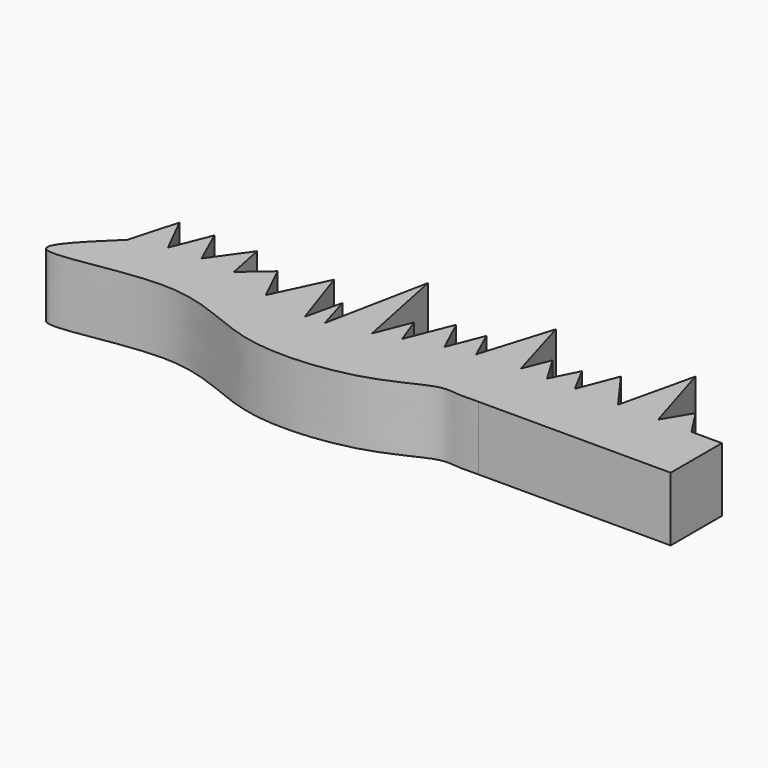
from build123d import *

# Parameters (mm, degrees)
F1_DEPTH = 12.7


# Not quite as in the source:
# - a feature names something its author has since deleted; it is built from what else it names


with BuildPart() as f1:
    # F0 (on Top) → F1 (new body)
    with BuildSketch(Plane.XY):
        with BuildLine():
            Line((29.1566601902, 1.7817904405), (29.1566601902, 14.4817904405))
            Line((29.1566601902, 14.4817904405), (23.1322348118, 14.4817904405))
            Line((23.1322348118, 14.4817904405), (16.5050514042, 14.4817904405))
            Line((16.5050514042, 14.4817904405), (8.552428335, 14.4817904405))
            Line((8.552428335, 14.4817904405), (0, 14.4817904405))
            Line((0, 14.4817904405), (-5.4972041398, 14.4817904405))
            Line((-5.4972041398, 14.4817904405), (-8.9433398098, 14.4817904405))
            add(Edge.make_bspline(
                [(-8.9433398098, 14.4817904405), (-10.7573023584, 14.5540929372), (-13.6536245903, 14.6695370673), (-17.5443018447, 14.2319983354), (-19.1478505954, 13.9692945078)],
                knots=[0, 0, 0, 0, 0.1219531365, 0.1947204372, 0.1947204372, 0.1947204372, 0.1947204372], degree=3))
            add(Edge.make_bspline(
                [(-19.1478505954, 13.9692945078), (-20.7855145388, 13.7010017066), (-22.5792086961, 13.3292483099), (-24.5403655562, 12.8306326712)],
                knots=[0.1947204372, 0.1947204372, 0.1947204372, 0.1947204372, 0.2690358483, 0.2690358483, 0.2690358483, 0.2690358483], degree=3))
            add(Edge.make_bspline(
                [(-24.5403655562, 12.8306326712), (-25.4054556528, 12.6106872606), (-27.5608275588, 12.0233152228), (-29.9097113738, 11.2820530364), (-31.3234997305, 10.8352217448)],
                knots=[0.2690358483, 0.2690358483, 0.2690358483, 0.2690358483, 0.3018172782, 0.3477460441, 0.3477460441, 0.3477460441, 0.3477460441], degree=3))
            add(Edge.make_bspline(
                [(-31.3234997305, 10.8352217448), (-32.8813721767, 10.3428523218), (-34.4916669077, 9.8331294404), (-36.1239915531, 9.3570380081)],
                knots=[0.3477460441, 0.3477460441, 0.3477460441, 0.3477460441, 0.3983555703, 0.3983555703, 0.3983555703, 0.3983555703], degree=3))
            add(Edge.make_bspline(
                [(-36.1239915531, 9.3570380081), (-38.7371673177, 8.5948669557), (-41.406802576, 7.9188884572), (-44.0082018162, 7.5382862352)],
                knots=[0.3983555703, 0.3983555703, 0.3983555703, 0.3983555703, 0.4793759651, 0.4793759651, 0.4793759651, 0.4793759651], degree=3))
            add(Edge.make_bspline(
                [(-44.0082018162, 7.5382862352), (-45.2733883847, 7.3531809228), (-46.5224347573, 7.2379423921), (-47.7409961664, 7.2166347961)],
                knots=[0.4793759651, 0.4793759651, 0.4793759651, 0.4793759651, 0.518780111, 0.518780111, 0.518780111, 0.518780111], degree=3))
            add(Edge.make_bspline(
                [(-47.7409961664, 7.2166347961), (-48.61023628, 7.2014353839), (-51.8736517816, 7.3260381182), (-54.8343256873, 8.2766625789), (-57.0016363215, 9.090849647)],
                knots=[0.518780111, 0.518780111, 0.518780111, 0.518780111, 0.5468883902, 0.6262253297, 0.6262253297, 0.6262253297, 0.6262253297], degree=3))
            add(Edge.make_bspline(
                [(-57.0016363215, 9.090849647), (-59.8222284032, 10.150452992), (-62.6109209229, 11.4001772385), (-65.6900354035, 12.0947333053)],
                knots=[0.6262253297, 0.6262253297, 0.6262253297, 0.6262253297, 0.7294764002, 0.7294764002, 0.7294764002, 0.7294764002], degree=3))
            add(Edge.make_bspline(
                [(-65.6900354035, 12.0947333053), (-67.0336130762, 12.397804214), (-69.2092078019, 12.7047556683), (-71.5833285763, 12.6062540598), (-72.4382368268, 12.5328440974)],
                knots=[0.7294764002, 0.7294764002, 0.7294764002, 0.7294764002, 0.7745302084, 0.7995461596, 0.7995461596, 0.7995461596, 0.7995461596], degree=3))
            add(Edge.make_bspline(
                [(-72.4382368268, 12.5328440974), (-78.4000977285, 12.0209061386), (-85.6590909795, 9.2956107983), (-85.3310582144, 10.1307918098), (-85.2885097265, 10.2391215041)],
                knots=[0.7995461596, 0.7995461596, 0.7995461596, 0.7995461596, 0.9739995247, 1, 1, 1, 1], degree=3))
            add(Edge.make_bspline(
                [(-8.9433398098, 1.7817904405), (-10.3062057468, 1.7346839959), (-12.9857258176, 1.6420683833), (-17.1466296289, 2.4827049446), (-27.1606442527, -4.0355858357), (-51.6393795509, -6.6773487114), (-67.5806364014, 5.6865791664), (-100.6765031612, -4.5794896544), (-89.9229154748, 5.7761967552), (-85.2885097265, 10.2391215041)],
                knots=[0, 0, 0, 0, 0.0795605261, 0.1564233287, 0.2898559981, 0.4816905838, 0.6666516763, 0.8563389789, 1, 1, 1, 1], degree=3))
            Line((-8.9433398098, 1.7817904405), (29.1566601902, 1.7817904405))
        make_face()
        with BuildLine():
            Line((-82.6221928, 19.7822675109), (-85.2885097265, 10.2391215041))
            add(Edge.make_bspline(
                [(-72.4382368268, 12.5328440974), (-78.4000977285, 12.0209061386), (-85.6590909795, 9.2956107983), (-85.3310582144, 10.1307918098), (-85.2885097265, 10.2391215041)],
                knots=[0.7995461596, 0.7995461596, 0.7995461596, 0.7995461596, 0.9739995247, 1, 1, 1, 1], degree=3))
            Line((-72.4382368268, 12.5328440974), (-75.7119506598, 19.7822675109))
            Line((-75.7119506598, 19.7822675109), (-78.7689969505, 12.0947333053))
            Line((-78.7689969505, 12.0947333053), (-82.6221928, 19.7822675109))
        make_face()
        with BuildLine():
            Line((-67.2413259745, 19.7822675109), (-72.4382368268, 12.5328440974))
            add(Edge.make_bspline(
                [(-65.6900354035, 12.0947333053), (-67.0336130762, 12.397804214), (-69.2092078019, 12.7047556683), (-71.5833285763, 12.6062540598), (-72.4382368268, 12.5328440974)],
                knots=[0.7294764002, 0.7294764002, 0.7294764002, 0.7294764002, 0.7745302084, 0.7995461596, 0.7995461596, 0.7995461596, 0.7995461596], degree=3))
            Line((-65.6900354035, 12.0947333053), (-67.2413259745, 19.7822675109))
        make_face()
        with BuildLine():
            Line((-51.9719198346, 19.7822675109), (-57.0016363215, 9.090849647))
            add(Edge.make_bspline(
                [(-47.7409961664, 7.2166347961), (-48.61023628, 7.2014353839), (-51.8736517816, 7.3260381182), (-54.8343256873, 8.2766625789), (-57.0016363215, 9.090849647)],
                knots=[0.518780111, 0.518780111, 0.518780111, 0.518780111, 0.5468883902, 0.6262253297, 0.6262253297, 0.6262253297, 0.6262253297], degree=3))
            Line((-47.7409961664, 7.2166347961), (-51.9719198346, 19.7822675109))
        make_face()
        with BuildLine():
            Line((-46.0647791624, 14.4817904405), (-47.7409961664, 7.2166347961))
            add(Edge.make_bspline(
                [(-44.0082018162, 7.5382862352), (-45.2733883847, 7.3531809228), (-46.5224347573, 7.2379423921), (-47.7409961664, 7.2166347961)],
                knots=[0.4793759651, 0.4793759651, 0.4793759651, 0.4793759651, 0.518780111, 0.518780111, 0.518780111, 0.518780111], degree=3))
            Line((-44.0082018162, 7.5382862352), (-46.0647791624, 14.4817904405))
        make_face()
        with BuildLine():
            Line((-39.9164316104, 27.9997758427), (-44.0082018162, 7.5382862352))
            add(Edge.make_bspline(
                [(-36.1239915531, 9.3570380081), (-38.7371673177, 8.5948669557), (-41.406802576, 7.9188884572), (-44.0082018162, 7.5382862352)],
                knots=[0.3983555703, 0.3983555703, 0.3983555703, 0.3983555703, 0.4793759651, 0.4793759651, 0.4793759651, 0.4793759651], degree=3))
            Line((-36.1239915531, 9.3570380081), (-39.9164316104, 27.9997758427))
        make_face()
        with BuildLine():
            Line((-33.3588495851, 16.3105223328), (-36.1239915531, 9.3570380081))
            add(Edge.make_bspline(
                [(-31.3234997305, 10.8352217448), (-32.8813721767, 10.3428523218), (-34.4916669077, 9.8331294404), (-36.1239915531, 9.3570380081)],
                knots=[0.3477460441, 0.3477460441, 0.3477460441, 0.3477460441, 0.3983555703, 0.3983555703, 0.3983555703, 0.3983555703], degree=3))
            Line((-31.3234997305, 10.8352217448), (-33.3588495851, 16.3105223328))
        make_face()
        with BuildLine():
            add(Edge.make_bspline(
                [(-24.5403655562, 12.8306326712), (-25.4054556528, 12.6106872606), (-27.5608275588, 12.0233152228), (-29.9097113738, 11.2820530364), (-31.3234997305, 10.8352217448)],
                knots=[0.2690358483, 0.2690358483, 0.2690358483, 0.2690358483, 0.3018172782, 0.3477460441, 0.3477460441, 0.3477460441, 0.3477460441], degree=3))
            Line((-24.5403655562, 12.8306326712), (-27.7655925602, 19.7822675109))
            Line((-27.7655925602, 19.7822675109), (-31.3234997305, 10.8352217448))
        make_face()
        with BuildLine():
            add(Edge.make_bspline(
                [(-19.1478505954, 13.9692945078), (-20.7855145388, 13.7010017066), (-22.5792086961, 13.3292483099), (-24.5403655562, 12.8306326712)],
                knots=[0.1947204372, 0.1947204372, 0.1947204372, 0.1947204372, 0.2690358483, 0.2690358483, 0.2690358483, 0.2690358483], degree=3))
            Line((-19.1478505954, 13.9692945078), (-21.7759590596, 19.7822675109))
            Line((-21.7759590596, 19.7822675109), (-24.5403655562, 12.8306326712))
        make_face()
        Polygon((-5.4972041398, 14.4817904405), (0, 14.4817904405), (-2.846329473, 19.7822675109), align=None)
        Polygon((0, 14.4817904405), (8.552428335, 14.4817904405), (2.9855933972, 22.1680551767), align=None)
        Polygon((8.552428335, 14.4817904405), (16.5050514042, 14.4817904405), (11.9985649362, 29.325414449), align=None)
        Polygon((16.5050514042, 14.4817904405), (23.1322348118, 14.4817904405), (19.6860991418, 19.7822675109), align=None)
        with BuildLine():
            Line((-8.9433398098, 14.4817904405), (-5.4972041398, 14.4817904405))
            Line((-5.4972041398, 14.4817904405), (-8.6782518774, 19.7822675109))
            Line((-8.6782518774, 19.7822675109), (-10.7573023584, 14.5540929372))
            Line((-10.7573023584, 14.5540929372), (-14.7752631456, 28.2258577645))
            Line((-14.7752631456, 28.2258577645), (-19.1478505954, 13.9692945078))
            add(Edge.make_bspline(
                [(-8.9433398098, 14.4817904405), (-10.7573023584, 14.5540929372), (-13.6536245903, 14.6695370673), (-17.5443018447, 14.2319983354), (-19.1478505954, 13.9692945078)],
                knots=[0, 0, 0, 0, 0.1219531365, 0.1947204372, 0.1947204372, 0.1947204372, 0.1947204372], degree=3))
        make_face()
        with BuildLine():
            Line((-60.5539940298, 16.5334325284), (-65.6900354035, 12.0947333053))
            add(Edge.make_bspline(
                [(-57.0016363215, 9.090849647), (-59.8222284032, 10.150452992), (-62.6109209229, 11.4001772385), (-65.6900354035, 12.0947333053)],
                knots=[0.6262253297, 0.6262253297, 0.6262253297, 0.6262253297, 0.7294764002, 0.7294764002, 0.7294764002, 0.7294764002], degree=3))
            Line((-57.0016363215, 9.090849647), (-60.5539940298, 16.5334325284))
        make_face()
    extrude(amount=F1_DEPTH)


solid = f1.part
